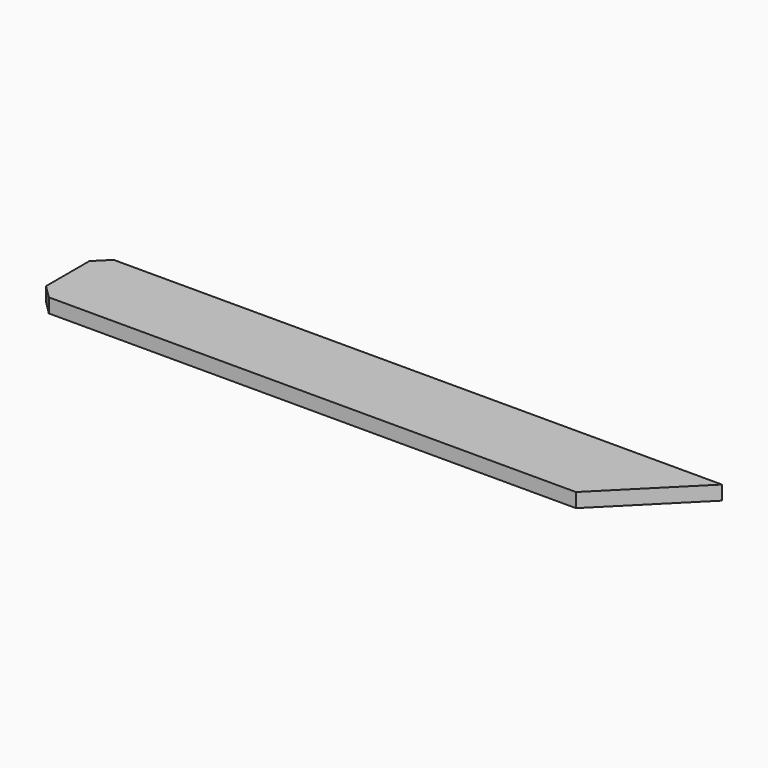
from build123d import *

# Parameters (mm, degrees)
F0_W     = 920
F0_H     = 120
F1_DEPTH = 21
F2_SIZE  = 20
F3_SIZE  = 119.99999


# Not quite as in the source:
# - a fillet or chamfer is up to 0.001 mm smaller than in the source, because OpenCascade refuses the exact size


with BuildPart() as f1:
    # F0 (on Top) → F1 (new body)
    with BuildSketch(Plane.XY):
        Rectangle(F0_W, F0_H)
    extrude(amount=F1_DEPTH)

    # F2
    f2_edges = [f1.edges().sort_by_distance(p)[0] for p in [
        (-460, 60, 10.5),
        (-460, -60, 10.5),
    ]]
    chamfer(f2_edges, length=F2_SIZE)

    # F3 (size 120 in the source; OpenCascade refuses exactly that, so slightly less here)
    f3_edges = [f1.edges().sort_by_distance(p)[0] for p in [
        (460, -60, 10.5),
    ]]
    chamfer(f3_edges, length=F3_SIZE)


solid = f1.part
